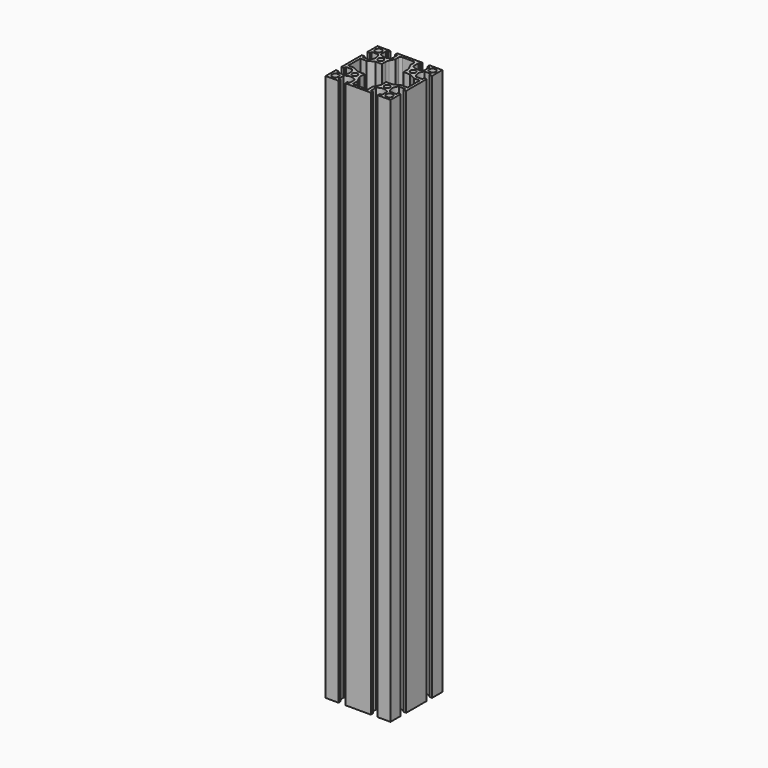
from build123d import *

# Parameters (mm, degrees)
F0_R     = 3
F0_R_2   = 2.5
F1_DEPTH = 507
F2_R     = 2
F3_R     = 7


# Not quite as in the source:
# - a feature names something its author has since deleted; it is built from what else it names


with BuildPart() as f1:
    # F0 (on Top) → F1 (new body)
    with BuildSketch(Plane.XY):
        with BuildLine():
            Line((18.15, -30), (30, -30))
            Line((30, -30), (30, -18.15))
            Line((30, -18.15), (27.5, -18.15))
            Line((27.5, -18.15), (27.5, -20.15))
            Line((27.5, -20.15), (21.5477069044, -20.15))
            ThreePointArc((21.5477069044, -20.15), (19.5, -15), (21.5477069044, -9.85))
            Line((21.5477069044, -9.85), (27.5, -9.85))
            Line((27.5, -9.85), (27.5, -11.85))
            Line((27.5, -11.85), (30, -11.85))
            Line((30, -11.85), (30, 11.85))
            Line((30, 11.85), (27.5, 11.85))
            Line((27.5, 11.85), (27.5, 9.85))
            Line((27.5, 9.85), (21.5477069044, 9.85))
            ThreePointArc((21.5477069044, 9.85), (19.5, 15), (21.5477069044, 20.15))
            Line((21.5477069044, 20.15), (27.5, 20.15))
            Line((27.5, 20.15), (27.5, 18.15))
            Line((27.5, 18.15), (30, 18.15))
            Line((30, 18.15), (30, 30))
            Line((30, 30), (18.15, 30))
            Line((18.15, 30), (18.15, 27.5))
            Line((18.15, 27.5), (20.15, 27.5))
            Line((20.15, 27.5), (20.15, 21.5477069044))
            ThreePointArc((20.15, 21.5477069044), (15, 19.5), (9.85, 21.5477069044))
            Line((9.85, 21.5477069044), (9.85, 27.5))
            Line((9.85, 27.5), (11.85, 27.5))
            Line((11.85, 27.5), (11.85, 30))
            Line((11.85, 30), (-11.85, 30))
            Line((-11.85, 30), (-11.85, 27.5))
            Line((-11.85, 27.5), (-9.85, 27.5))
            Line((-9.85, 27.5), (-9.85, 21.5477069044))
            ThreePointArc((-9.85, 21.5477069044), (-15, 19.5), (-20.15, 21.5477069044))
            Line((-20.15, 21.5477069044), (-20.15, 27.5))
            Line((-20.15, 27.5), (-18.15, 27.5))
            Line((-18.15, 27.5), (-18.15, 30))
            Line((-18.15, 30), (-30, 30))
            Line((-30, 30), (-30, 18.15))
            Line((-30, 18.15), (-27.5, 18.15))
            Line((-27.5, 18.15), (-27.5, 20.15))
            Line((-27.5, 20.15), (-21.5477069044, 20.15))
            ThreePointArc((-21.5477069044, 20.15), (-19.5, 15), (-21.5477069044, 9.85))
            Line((-21.5477069044, 9.85), (-27.5, 9.85))
            Line((-27.5, 9.85), (-27.5, 11.85))
            Line((-27.5, 11.85), (-30, 11.85))
            Line((-30, 11.85), (-30, -11.85))
            Line((-30, -11.85), (-27.5, -11.85))
            Line((-27.5, -11.85), (-27.5, -9.85))
            Line((-27.5, -9.85), (-21.5477069044, -9.85))
            ThreePointArc((-21.5477069044, -9.85), (-19.5, -15), (-21.5477069044, -20.15))
            Line((-21.5477069044, -20.15), (-27.5, -20.15))
            Line((-27.5, -20.15), (-27.5, -18.15))
            Line((-27.5, -18.15), (-30, -18.15))
            Line((-30, -18.15), (-30, -30))
            Line((-30, -30), (-18.15, -30))
            Line((-18.15, -30), (-18.15, -27.5))
            Line((-18.15, -27.5), (-20.15, -27.5))
            Line((-20.15, -27.5), (-20.15, -21.5477069044))
            ThreePointArc((-20.15, -21.5477069044), (-15, -19.5), (-9.85, -21.5477069044))
            Line((-9.85, -21.5477069044), (-9.85, -27.5))
            Line((-9.85, -27.5), (-11.85, -27.5))
            Line((-11.85, -27.5), (-11.85, -30))
            Line((-11.85, -30), (11.85, -30))
            Line((11.85, -30), (11.85, -27.5))
            Line((11.85, -27.5), (9.85, -27.5))
            Line((9.85, -27.5), (9.85, -21.5477069044))
            ThreePointArc((9.85, -21.5477069044), (15, -19.5), (20.15, -21.5477069044))
            Line((20.15, -21.5477069044), (20.15, -27.5))
            Line((20.15, -27.5), (18.15, -27.5))
            Line((18.15, -27.5), (18.15, -30))
        make_face()
        with Locations((-25, -25)):
            Circle(F0_R, mode=Mode.SUBTRACT)
        with Locations((-15, -15)):
            Circle(F0_R_2, mode=Mode.SUBTRACT)
        with Locations((25, -25)):
            Circle(F0_R, mode=Mode.SUBTRACT)
        with Locations((15, -15)):
            Circle(F0_R_2, mode=Mode.SUBTRACT)
        with Locations((-25, 25)):
            Circle(F0_R, mode=Mode.SUBTRACT)
        with Locations((-15, 15)):
            Circle(F0_R_2, mode=Mode.SUBTRACT)
        Polygon((-7, 22), (-7, 27.5), (0, 27.5), (7, 27.5), (7, 22), (10, 16), (10, 10), (16, 10), (22, 7), (27.5, 7), (27.5, 0), (27.5, -7), (22, -7), (16, -10), (10, -10), (10, -16), (7, -22), (7, -27.5), (0, -27.5), (-7, -27.5), (-7, -22), (-10, -16), (-10, -10), (-16, -10), (-22, -7), (-27.5, -7), (-27.5, 0), (-27.5, 7), (-22, 7), (-16, 10), (-10, 10), (-10, 16), align=None, mode=Mode.SUBTRACT)
        with Locations((15, 15)):
            Circle(F0_R_2, mode=Mode.SUBTRACT)
        with Locations((25, 25)):
            Circle(F0_R, mode=Mode.SUBTRACT)
    extrude(amount=F1_DEPTH)

    # F2
    f2_edges = [f1.edges().sort_by_distance(p)[0] for p in [
        (-7, 27.5, 253.5),
        (7, 27.5, 253.5),
    ]]
    fillet(f2_edges, radius=F2_R)

    # F3
    f3_edges = [f1.edges().sort_by_distance(p)[0] for p in [
        (-10, 16, 253.5),
        (10, 16, 253.5),
    ]]
    fillet(f3_edges, radius=F3_R)


solid = f1.part
